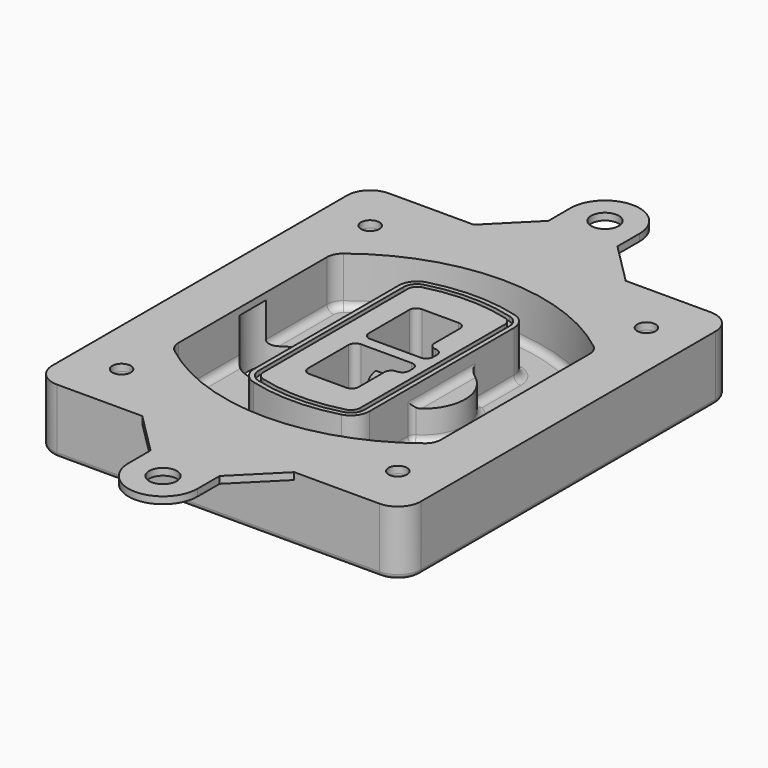
from build123d import *

# Parameters (mm, degrees)
F0_R      = 4
F1_DEPTH  = 25
F2_DEPTH  = 3
F3_DEPTH  = 18
F5_DEPTH  = 21
F6_DEPTH  = 2
F8_DEPTH  = 20
F9_DEPTH  = 16
F10_DEPTH = 25
F7_R      = 6
F7_R_2    = 4
F11_DEPTH = 6
F13_DEPTH = 9
F14_R     = 3
F15_R     = 2
F16_R     = 4
F16_R_2   = 6
F17_DEPTH = 3


# Not quite as in the source:
# - a feature names something its author has since deleted; it is built from what else it names


with BuildPart() as f1:
    # F0 (on Top) → F1 (new body)
    with BuildSketch(Plane.XY):
        with BuildLine():
            ThreePointArc((-80, -80), (-77.0710678119, -87.0710678119), (-70, -90))
            Line((-70, -90), (70, -90))
            ThreePointArc((70, -90), (77.0710678119, -87.0710678119), (80, -80))
            Line((80, -80), (80, 80))
            ThreePointArc((80, 80), (77.0710678119, 87.0710678119), (70, 90))
            Line((70, 90), (-70, 90))
            ThreePointArc((-70, 90), (-77.0710678119, 87.0710678119), (-80, 80))
            Line((-80, 80), (-80, -80))
        make_face()
        with Locations((-60, -67.5)):
            Circle(F0_R, mode=Mode.SUBTRACT)
        with Locations((60, -67.5)):
            Circle(F0_R, mode=Mode.SUBTRACT)
        with Locations((-60, 67.5)):
            Circle(F0_R, mode=Mode.SUBTRACT)
        with BuildLine():
            ThreePointArc((-64, 40.2934422872), (-62.5820384798, 46.4328484224), (-58.6153846154, 51.3286200352))
            ThreePointArc((-58.6153846154, 51.3286200352), (0, 71.5), (58.6153846154, 51.3286200352))
            ThreePointArc((58.6153846154, 51.3286200352), (62.5820384798, 46.4328484224), (64, 40.2934422872))
            Line((64, 40.2934422872), (64, -40.2934422872))
            ThreePointArc((64, -40.2934422872), (62.5820384798, -46.4328484224), (58.6153846154, -51.3286200352))
            ThreePointArc((58.6153846154, -51.3286200352), (0, -71.5), (-58.6153846154, -51.3286200352))
            ThreePointArc((-58.6153846154, -51.3286200352), (-62.5820384798, -46.4328484224), (-64, -40.2934422872))
            Line((-64, -40.2934422872), (-64, 40.2934422872))
        make_face(mode=Mode.SUBTRACT)
        with Locations((60, 67.5)):
            Circle(F0_R, mode=Mode.SUBTRACT)
        with BuildLine():
            ThreePointArc((58.6153846154, 51.3286200352), (0, 71.5), (-58.6153846154, 51.3286200352))
            ThreePointArc((-58.6153846154, 51.3286200352), (-62.5820384798, 46.4328484224), (-64, 40.2934422872))
            Line((-64, 40.2934422872), (-64, -40.2934422872))
            ThreePointArc((-64, -40.2934422872), (-62.5820384798, -46.4328484224), (-58.6153846154, -51.3286200352))
            ThreePointArc((-58.6153846154, -51.3286200352), (0, -71.5), (58.6153846154, -51.3286200352))
            ThreePointArc((58.6153846154, -51.3286200352), (62.5820384798, -46.4328484224), (64, -40.2934422872))
            Line((64, -40.2934422872), (64, 40.2934422872))
            ThreePointArc((64, 40.2934422872), (62.5820384798, 46.4328484224), (58.6153846154, 51.3286200352))
        make_face()
        with BuildLine():
            Line((-60, -40.2934422872), (-60, 40.2934422872))
            ThreePointArc((-60, 40.2934422872), (-58.9871703427, 44.6787323838), (-56.1538461538, 48.1757121072))
            ThreePointArc((-56.1538461538, 48.1757121072), (0, 67.5), (56.1538461538, 48.1757121072))
            ThreePointArc((56.1538461538, 48.1757121072), (58.9871703427, 44.6787323838), (60, 40.2934422872))
            Line((60, 40.2934422872), (60, -40.2934422872))
            ThreePointArc((60, -40.2934422872), (58.9871703427, -44.6787323838), (56.1538461538, -48.1757121072))
            ThreePointArc((56.1538461538, -48.1757121072), (0, -67.5), (-56.1538461538, -48.1757121072))
            ThreePointArc((-56.1538461538, -48.1757121072), (-58.9871703427, -44.6787323838), (-60, -40.2934422872))
        make_face(mode=Mode.SUBTRACT)
        with BuildLine():
            ThreePointArc((-56.1538461538, 48.1757121072), (-58.9871703427, 44.6787323838), (-60, 40.2934422872))
            Line((-60, 40.2934422872), (-60, -40.2934422872))
            ThreePointArc((-60, -40.2934422872), (-58.9871703427, -44.6787323838), (-56.1538461538, -48.1757121072))
            ThreePointArc((-56.1538461538, -48.1757121072), (0, -67.5), (56.1538461538, -48.1757121072))
            ThreePointArc((56.1538461538, -48.1757121072), (58.9871703427, -44.6787323838), (60, -40.2934422872))
            Line((60, -40.2934422872), (60, 40.2934422872))
            ThreePointArc((60, 40.2934422872), (58.9871703427, 44.6787323838), (56.1538461538, 48.1757121072))
            ThreePointArc((56.1538461538, 48.1757121072), (0, 67.5), (-56.1538461538, 48.1757121072))
        make_face()
        with BuildLine():
            ThreePointArc((54.3076923077, 45.8110311612), (56.2910192399, 43.3631453548), (57, 40.2934422872))
            Line((57, 40.2934422872), (57, -40.2934422872))
            ThreePointArc((57, -40.2934422872), (56.2910192399, -43.3631453548), (54.3076923077, -45.8110311612))
            ThreePointArc((54.3076923077, -45.8110311612), (0, -64.5), (-54.3076923077, -45.8110311612))
            ThreePointArc((-54.3076923077, -45.8110311612), (-56.2910192399, -43.3631453548), (-57, -40.2934422872))
            Line((-57, -40.2934422872), (-57, 40.2934422872))
            ThreePointArc((-57, 40.2934422872), (-56.2910192399, 43.3631453548), (-54.3076923077, 45.8110311612))
            ThreePointArc((-54.3076923077, 45.8110311612), (0, 64.5), (54.3076923077, 45.8110311612))
        make_face(mode=Mode.SUBTRACT)
        with BuildLine():
            Line((57, -40.2934422872), (57, 40.2934422872))
            ThreePointArc((57, 40.2934422872), (56.2910192399, 43.3631453548), (54.3076923077, 45.8110311612))
            ThreePointArc((54.3076923077, 45.8110311612), (0, 64.5), (-54.3076923077, 45.8110311612))
            ThreePointArc((-54.3076923077, 45.8110311612), (-56.2910192399, 43.3631453548), (-57, 40.2934422872))
            Line((-57, 40.2934422872), (-57, -40.2934422872))
            ThreePointArc((-57, -40.2934422872), (-56.2910192399, -43.3631453548), (-54.3076923077, -45.8110311612))
            ThreePointArc((-54.3076923077, -45.8110311612), (0, -64.5), (54.3076923077, -45.8110311612))
            ThreePointArc((54.3076923077, -45.8110311612), (56.2910192399, -43.3631453548), (57, -40.2934422872))
        make_face()
    extrude(amount=-F1_DEPTH)

    # F0 (on Top) → F2 (join)
    with BuildSketch(Plane.XY):
        with BuildLine():
            ThreePointArc((-56.1538461538, 48.1757121072), (-58.9871703427, 44.6787323838), (-60, 40.2934422872))
            Line((-60, 40.2934422872), (-60, -40.2934422872))
            ThreePointArc((-60, -40.2934422872), (-58.9871703427, -44.6787323838), (-56.1538461538, -48.1757121072))
            ThreePointArc((-56.1538461538, -48.1757121072), (0, -67.5), (56.1538461538, -48.1757121072))
            ThreePointArc((56.1538461538, -48.1757121072), (58.9871703427, -44.6787323838), (60, -40.2934422872))
            Line((60, -40.2934422872), (60, 40.2934422872))
            ThreePointArc((60, 40.2934422872), (58.9871703427, 44.6787323838), (56.1538461538, 48.1757121072))
            ThreePointArc((56.1538461538, 48.1757121072), (0, 67.5), (-56.1538461538, 48.1757121072))
        make_face()
        with BuildLine():
            ThreePointArc((54.3076923077, 45.8110311612), (56.2910192399, 43.3631453548), (57, 40.2934422872))
            Line((57, 40.2934422872), (57, -40.2934422872))
            ThreePointArc((57, -40.2934422872), (56.2910192399, -43.3631453548), (54.3076923077, -45.8110311612))
            ThreePointArc((54.3076923077, -45.8110311612), (0, -64.5), (-54.3076923077, -45.8110311612))
            ThreePointArc((-54.3076923077, -45.8110311612), (-56.2910192399, -43.3631453548), (-57, -40.2934422872))
            Line((-57, -40.2934422872), (-57, 40.2934422872))
            ThreePointArc((-57, 40.2934422872), (-56.2910192399, 43.3631453548), (-54.3076923077, 45.8110311612))
            ThreePointArc((-54.3076923077, 45.8110311612), (0, 64.5), (54.3076923077, 45.8110311612))
        make_face(mode=Mode.SUBTRACT)
    extrude(amount=F2_DEPTH)

    # F0 (on Top) → F3 (cut)
    with BuildSketch(Plane.XY):
        with BuildLine():
            Line((57, -40.2934422872), (57, 40.2934422872))
            ThreePointArc((57, 40.2934422872), (56.2910192399, 43.3631453548), (54.3076923077, 45.8110311612))
            ThreePointArc((54.3076923077, 45.8110311612), (0, 64.5), (-54.3076923077, 45.8110311612))
            ThreePointArc((-54.3076923077, 45.8110311612), (-56.2910192399, 43.3631453548), (-57, 40.2934422872))
            Line((-57, 40.2934422872), (-57, -40.2934422872))
            ThreePointArc((-57, -40.2934422872), (-56.2910192399, -43.3631453548), (-54.3076923077, -45.8110311612))
            ThreePointArc((-54.3076923077, -45.8110311612), (0, -64.5), (54.3076923077, -45.8110311612))
            ThreePointArc((54.3076923077, -45.8110311612), (56.2910192399, -43.3631453548), (57, -40.2934422872))
        make_face()
    extrude(amount=-F3_DEPTH, mode=Mode.SUBTRACT)

    # F4 (on face) → F5 (join, through all)
    with BuildSketch(Plane.XY.offset(3)):
        with BuildLine():
            ThreePointArc((-25, -39.2465276821), (-23.3511545998, -44.1109737193), (-19.0842911877, -46.9702398883))
            ThreePointArc((-19.0842911877, -46.9702398883), (0, -49.5), (19.0842911877, -46.9702398883))
            ThreePointArc((19.0842911877, -46.9702398883), (23.3511545998, -44.1109737193), (25, -39.2465276821))
            Line((25, -39.2465276821), (25, 39.2465276821))
            ThreePointArc((25, 39.2465276821), (23.3511545998, 44.1109737193), (19.0842911877, 46.9702398883))
            ThreePointArc((19.0842911877, 46.9702398883), (0, 49.5), (-19.0842911877, 46.9702398883))
            ThreePointArc((-19.0842911877, 46.9702398883), (-23.3511545998, 44.1109737193), (-25, 39.2465276821))
            Line((-25, 39.2465276821), (-25, -39.2465276821))
        make_face()
        with BuildLine():
            ThreePointArc((18.5632183908, 45.0393118368), (21.7633659499, 42.89486221), (23, 39.2465276821))
            Line((23, 39.2465276821), (23, -39.2465276821))
            ThreePointArc((23, -39.2465276821), (21.7633659499, -42.89486221), (18.5632183908, -45.0393118368))
            ThreePointArc((18.5632183908, -45.0393118368), (0, -47.5), (-18.5632183908, -45.0393118368))
            ThreePointArc((-18.5632183908, -45.0393118368), (-21.7633659499, -42.89486221), (-23, -39.2465276821))
            Line((-23, -39.2465276821), (-23, 39.2465276821))
            ThreePointArc((-23, 39.2465276821), (-21.7633659499, 42.89486221), (-18.5632183908, 45.0393118368))
            ThreePointArc((-18.5632183908, 45.0393118368), (0, 47.5), (18.5632183908, 45.0393118368))
        make_face(mode=Mode.SUBTRACT)
        with BuildLine():
            Line((23, -39.2465276821), (23, 39.2465276821))
            ThreePointArc((23, 39.2465276821), (21.7633659499, 42.89486221), (18.5632183908, 45.0393118368))
            ThreePointArc((18.5632183908, 45.0393118368), (0, 47.5), (-18.5632183908, 45.0393118368))
            ThreePointArc((-18.5632183908, 45.0393118368), (-21.7633659499, 42.89486221), (-23, 39.2465276821))
            Line((-23, 39.2465276821), (-23, -39.2465276821))
            ThreePointArc((-23, -39.2465276821), (-21.7633659499, -42.89486221), (-18.5632183908, -45.0393118368))
            ThreePointArc((-18.5632183908, -45.0393118368), (0, -47.5), (18.5632183908, -45.0393118368))
            ThreePointArc((18.5632183908, -45.0393118368), (21.7633659499, -42.89486221), (23, -39.2465276821))
        make_face()
        with BuildLine():
            ThreePointArc((18.0421455939, 43.1083837852), (20.1755772999, 41.6787507007), (21, 39.2465276821))
            Line((21, 39.2465276821), (21, -39.2465276821))
            ThreePointArc((21, -39.2465276821), (20.1755772999, -41.6787507007), (18.0421455939, -43.1083837852))
            ThreePointArc((18.0421455939, -43.1083837852), (0, -45.5), (-18.0421455939, -43.1083837852))
            ThreePointArc((-18.0421455939, -43.1083837852), (-20.1755772999, -41.6787507007), (-21, -39.2465276821))
            Line((-21, -39.2465276821), (-21, 39.2465276821))
            ThreePointArc((-21, 39.2465276821), (-20.1755772999, 41.6787507007), (-18.0421455939, 43.1083837852))
            ThreePointArc((-18.0421455939, 43.1083837852), (0, 45.5), (18.0421455939, 43.1083837852))
        make_face(mode=Mode.SUBTRACT)
        with BuildLine():
            Line((21, -39.2465276821), (21, 39.2465276821))
            ThreePointArc((21, 39.2465276821), (20.1755772999, 41.6787507007), (18.0421455939, 43.1083837852))
            ThreePointArc((18.0421455939, 43.1083837852), (0, 45.5), (-18.0421455939, 43.1083837852))
            ThreePointArc((-18.0421455939, 43.1083837852), (-20.1755772999, 41.6787507007), (-21, 39.2465276821))
            Line((-21, 39.2465276821), (-21, -39.2465276821))
            ThreePointArc((-21, -39.2465276821), (-20.1755772999, -41.6787507007), (-18.0421455939, -43.1083837852))
            ThreePointArc((-18.0421455939, -43.1083837852), (0, -45.5), (18.0421455939, -43.1083837852))
            ThreePointArc((18.0421455939, -43.1083837852), (20.1755772999, -41.6787507007), (21, -39.2465276821))
        make_face()
        with BuildLine():
            Line((-8, -2.5), (14, -2.5))
            ThreePointArc((14, -2.5), (16.1213203436, -3.3786796564), (17, -5.5))
            Line((17, -5.5), (17, -7.5))
            ThreePointArc((17, -7.5), (16.1213203436, -9.6213203436), (14, -10.5))
            ThreePointArc((14, -10.5), (11.8786796564, -11.3786796564), (11, -13.5))
            Line((11, -13.5), (11, -27.5))
            ThreePointArc((11, -27.5), (10.1213203436, -29.6213203436), (8, -30.5))
            Line((8, -30.5), (-8, -30.5))
            ThreePointArc((-8, -30.5), (-10.1213203436, -29.6213203436), (-11, -27.5))
            Line((-11, -27.5), (-11, -5.5))
            ThreePointArc((-11, -5.5), (-10.1213203436, -3.3786796564), (-8, -2.5))
        make_face(mode=Mode.SUBTRACT)
        with BuildLine():
            ThreePointArc((-8, 2.5), (-10.1213203436, 3.3786796564), (-11, 5.5))
            Line((-11, 5.5), (-11, 27.5))
            ThreePointArc((-11, 27.5), (-10.1213203436, 29.6213203436), (-8, 30.5))
            Line((-8, 30.5), (8, 30.5))
            ThreePointArc((8, 30.5), (10.1213203436, 29.6213203436), (11, 27.5))
            Line((11, 27.5), (11, 13.5))
            ThreePointArc((11, 13.5), (11.8786796564, 11.3786796564), (14, 10.5))
            ThreePointArc((14, 10.5), (16.1213203436, 9.6213203436), (17, 7.5))
            Line((17, 7.5), (17, 5.5))
            ThreePointArc((17, 5.5), (16.1213203436, 3.3786796564), (14, 2.5))
            Line((14, 2.5), (-8, 2.5))
        make_face(mode=Mode.SUBTRACT)
    extrude(amount=-F5_DEPTH)

    # F4 (on face) → F6 (cut)
    with BuildSketch(Plane.XY.offset(3)):
        with BuildLine():
            Line((23, -39.2465276821), (23, 39.2465276821))
            ThreePointArc((23, 39.2465276821), (21.7633659499, 42.89486221), (18.5632183908, 45.0393118368))
            ThreePointArc((18.5632183908, 45.0393118368), (0, 47.5), (-18.5632183908, 45.0393118368))
            ThreePointArc((-18.5632183908, 45.0393118368), (-21.7633659499, 42.89486221), (-23, 39.2465276821))
            Line((-23, 39.2465276821), (-23, -39.2465276821))
            ThreePointArc((-23, -39.2465276821), (-21.7633659499, -42.89486221), (-18.5632183908, -45.0393118368))
            ThreePointArc((-18.5632183908, -45.0393118368), (0, -47.5), (18.5632183908, -45.0393118368))
            ThreePointArc((18.5632183908, -45.0393118368), (21.7633659499, -42.89486221), (23, -39.2465276821))
        make_face()
        with BuildLine():
            ThreePointArc((18.0421455939, 43.1083837852), (20.1755772999, 41.6787507007), (21, 39.2465276821))
            Line((21, 39.2465276821), (21, -39.2465276821))
            ThreePointArc((21, -39.2465276821), (20.1755772999, -41.6787507007), (18.0421455939, -43.1083837852))
            ThreePointArc((18.0421455939, -43.1083837852), (0, -45.5), (-18.0421455939, -43.1083837852))
            ThreePointArc((-18.0421455939, -43.1083837852), (-20.1755772999, -41.6787507007), (-21, -39.2465276821))
            Line((-21, -39.2465276821), (-21, 39.2465276821))
            ThreePointArc((-21, 39.2465276821), (-20.1755772999, 41.6787507007), (-18.0421455939, 43.1083837852))
            ThreePointArc((-18.0421455939, 43.1083837852), (0, 45.5), (18.0421455939, 43.1083837852))
        make_face(mode=Mode.SUBTRACT)
    extrude(amount=-F6_DEPTH, mode=Mode.SUBTRACT)

    # F7 (on face) → F8 (join)
    with BuildSketch(Plane(origin=(0, 0, -25), x_dir=(1, 0, 0), z_dir=(0, 0, -1))):
        with BuildLine():
            ThreePointArc((3.28842436, 0), (16.7567035675, 13.4682792075), (30.224982775, 0))
            Line((30.224982775, 0), (35.224982775, 0))
            ThreePointArc((35.224982775, 0), (16.7567035675, 18.4682792075), (-1.71157564, 0))
            Line((-1.71157564, 0), (3.28842436, 0))
        make_face()
        with BuildLine():
            Line((3.28842436, 0), (30.224982775, 0))
            ThreePointArc((30.224982775, 0), (16.7567035675, 13.4682792075), (3.28842436, 0))
        make_face()
        with BuildLine():
            ThreePointArc((3.28842436, 0), (16.7567035675, -13.4682792075), (30.224982775, 0))
            Line((30.224982775, 0), (3.28842436, 0))
        make_face()
        with BuildLine():
            Line((35.224982775, 0), (30.224982775, 0))
            ThreePointArc((30.224982775, 0), (16.7567035675, -13.4682792075), (3.28842436, 0))
            Line((3.28842436, 0), (-1.71157564, 0))
            ThreePointArc((-1.71157564, 0), (16.7567035675, -18.4682792075), (35.224982775, 0))
        make_face()
    extrude(amount=-F8_DEPTH)

    # F7 (on face) → F9 (cut)
    with BuildSketch(Plane(origin=(0, 0, -25), x_dir=(1, 0, 0), z_dir=(0, 0, -1))):
        with BuildLine():
            Line((3.28842436, 0), (30.224982775, 0))
            ThreePointArc((30.224982775, 0), (16.7567035675, 13.4682792075), (3.28842436, 0))
        make_face()
        with BuildLine():
            ThreePointArc((3.28842436, 0), (16.7567035675, -13.4682792075), (30.224982775, 0))
            Line((30.224982775, 0), (3.28842436, 0))
        make_face()
    extrude(amount=-F9_DEPTH, mode=Mode.SUBTRACT)

    # F7 (on face) → F10 (cut)
    with BuildSketch(Plane(origin=(0, 0, -25), x_dir=(1, 0, 0), z_dir=(0, 0, -1))):
        with BuildLine():
            Line((-59.0318229325, 0), (-32.0952645175, 0))
            ThreePointArc((-32.0952645175, 0), (-45.563543725, 13.4682792075), (-59.0318229325, 0))
        make_face()
        with BuildLine():
            ThreePointArc((-59.0318229325, 0), (-45.563543725, -13.4682792075), (-32.0952645175, 0))
            Line((-32.0952645175, 0), (-59.0318229325, 0))
        make_face()
    extrude(amount=-F10_DEPTH, mode=Mode.SUBTRACT)

    # F7 (on face) → F11 (cut)
    with BuildSketch(Plane(origin=(0, 0, -25), x_dir=(1, 0, 0), z_dir=(0, 0, -1))):
        with Locations((60, -67.5)):
            Circle(F7_R)
        with Locations((60, -67.5)):
            Circle(F7_R_2, mode=Mode.SUBTRACT)
        with Locations((-60, -67.5)):
            Circle(F7_R)
        with Locations((-60, -67.5)):
            Circle(F7_R_2, mode=Mode.SUBTRACT)
        with Locations((-60, 67.5)):
            Circle(F7_R)
        with Locations((-60, 67.5)):
            Circle(F7_R_2, mode=Mode.SUBTRACT)
        with Locations((60, 67.5)):
            Circle(F7_R)
        with Locations((60, 67.5)):
            Circle(F7_R_2, mode=Mode.SUBTRACT)
    extrude(amount=-F11_DEPTH, mode=Mode.SUBTRACT)

    # F12 (on face) → F13 (cut, through all)
    with BuildSketch(Plane(origin=(0, 0, -9), x_dir=(1, 0, 0), z_dir=(0, 0, -1))):
        with BuildLine():
            Line((11, 13.5), (11, 17.5481537753))
            ThreePointArc((11, 17.5481537753), (2.5696536419, 11.8239143813), (-1.5415842455, 2.5))
            Line((-1.5415842455, 2.5), (3.5224848595, 2.5))
            ThreePointArc((3.5224848595, 2.5), (6.1857188154, 8.3455872281), (11.2536447004, 12.2927168648))
            ThreePointArc((11.2536447004, 12.2927168648), (11.0640958889, 12.8831798879), (11, 13.5))
        make_face()
        with BuildLine():
            ThreePointArc((11.2536447004, -12.2927168648), (6.1857188154, -8.3455872281), (3.5224848595, -2.5))
            Line((3.5224848595, -2.5), (-1.5415842455, -2.5))
            ThreePointArc((-1.5415842455, -2.5), (2.5696536419, -11.8239143813), (11, -17.5481537753))
            Line((11, -17.5481537753), (11, -13.5))
            ThreePointArc((11, -13.5), (11.0640958889, -12.8831798879), (11.2536447004, -12.2927168648))
        make_face()
        with BuildLine():
            ThreePointArc((11.2536447004, 12.2927168648), (6.1857188154, 8.3455872281), (3.5224848595, 2.5))
            Line((3.5224848595, 2.5), (14, 2.5))
            ThreePointArc((14, 2.5), (16.1213203436, 3.3786796564), (17, 5.5))
            Line((17, 5.5), (17, 7.5))
            ThreePointArc((17, 7.5), (16.1213203436, 9.6213203436), (14, 10.5))
            ThreePointArc((14, 10.5), (12.3601599782, 10.9878446101), (11.2536447004, 12.2927168648))
        make_face()
        with BuildLine():
            Line((14, -2.5), (3.5224848595, -2.5))
            ThreePointArc((3.5224848595, -2.5), (6.1857188154, -8.3455872281), (11.2536447004, -12.2927168648))
            ThreePointArc((11.2536447004, -12.2927168648), (12.3601599782, -10.9878446101), (14, -10.5))
            ThreePointArc((14, -10.5), (16.1213203436, -9.6213203436), (17, -7.5))
            Line((17, -7.5), (17, -5.5))
            ThreePointArc((17, -5.5), (16.1213203436, -3.3786796564), (14, -2.5))
        make_face()
    extrude(amount=F13_DEPTH, mode=Mode.SUBTRACT)

    # F14
    f14_edges = [f1.edges().sort_by_distance(p)[0] for p in [
        (-57, -23.703476, -18),
        (-57, 23.703476, -18),
        (25, 0, -5),
        (25, 16.526506, -11.5),
        (25, -16.526506, -11.5),
        (25, -27.886517, -18),
        (35.224983, 0, -18),
    ]]
    fillet(f14_edges, radius=F14_R)

    # F15
    f15_edges = [f1.edges().sort_by_distance(p)[0] for p in [
        (0, -90, -25),
    ]]
    fillet(f15_edges, radius=F15_R)

    # F16 (on face) → F17 (join, through all)
    with BuildSketch(Plane.XY):
        with BuildLine():
            Line((33, 90), (-33, 90))
            Line((-33, 90), (-70, 90))
            ThreePointArc((-70, 90), (-77.0710678119, 87.0710678119), (-80, 80))
            Line((-80, 80), (-80, -80))
            ThreePointArc((-80, -80), (-77.0710678119, -87.0710678119), (-70, -90))
            Line((-70, -90), (-33, -90))
            Line((-33, -90), (33, -90))
            Line((33, -90), (70, -90))
            ThreePointArc((70, -90), (77.0710678119, -87.0710678119), (80, -80))
            Line((80, -80), (80, 80))
            ThreePointArc((80, 80), (77.0710678119, 87.0710678119), (70, 90))
            Line((70, 90), (33, 90))
        make_face()
        with Locations((-60, -67.5)):
            Circle(F16_R, mode=Mode.SUBTRACT)
        with Locations((60, -67.5)):
            Circle(F16_R, mode=Mode.SUBTRACT)
        with Locations((-60, 67.5)):
            Circle(F16_R, mode=Mode.SUBTRACT)
        with BuildLine():
            ThreePointArc((-60, 40.2934422872), (-58.9871703427, 44.6787323838), (-56.1538461538, 48.1757121072))
            ThreePointArc((-56.1538461538, 48.1757121072), (0, 67.5), (56.1538461538, 48.1757121072))
            ThreePointArc((56.1538461538, 48.1757121072), (58.9871703427, 44.6787323838), (60, 40.2934422872))
            Line((60, 40.2934422872), (60, -40.2934422872))
            ThreePointArc((60, -40.2934422872), (58.9871703427, -44.6787323838), (56.1538461538, -48.1757121072))
            ThreePointArc((56.1538461538, -48.1757121072), (0, -67.5), (-56.1538461538, -48.1757121072))
            ThreePointArc((-56.1538461538, -48.1757121072), (-58.9871703427, -44.6787323838), (-60, -40.2934422872))
            Line((-60, -40.2934422872), (-60, 40.2934422872))
        make_face(mode=Mode.SUBTRACT)
        with Locations((60, 67.5)):
            Circle(F16_R, mode=Mode.SUBTRACT)
        with BuildLine():
            Line((-15, 108), (-33, 90))
            Line((-33, 90), (33, 90))
            Line((33, 90), (15, 108))
            Line((15, 108), (15, 120))
            ThreePointArc((15, 120), (0, 135), (-15, 120))
            Line((-15, 120), (-15, 108))
        make_face()
        with Locations((0, 120)):
            Circle(F16_R_2, mode=Mode.SUBTRACT)
        with BuildLine():
            Line((33, -90), (-33, -90))
            Line((-33, -90), (-15, -108))
            Line((-15, -108), (-15, -120))
            ThreePointArc((-15, -120), (0, -135), (15, -120))
            Line((15, -120), (15, -108))
            Line((15, -108), (33, -90))
        make_face()
        with Locations((0, -120)):
            Circle(F16_R_2, mode=Mode.SUBTRACT)
    extrude(amount=F17_DEPTH)


solid = f1.part
